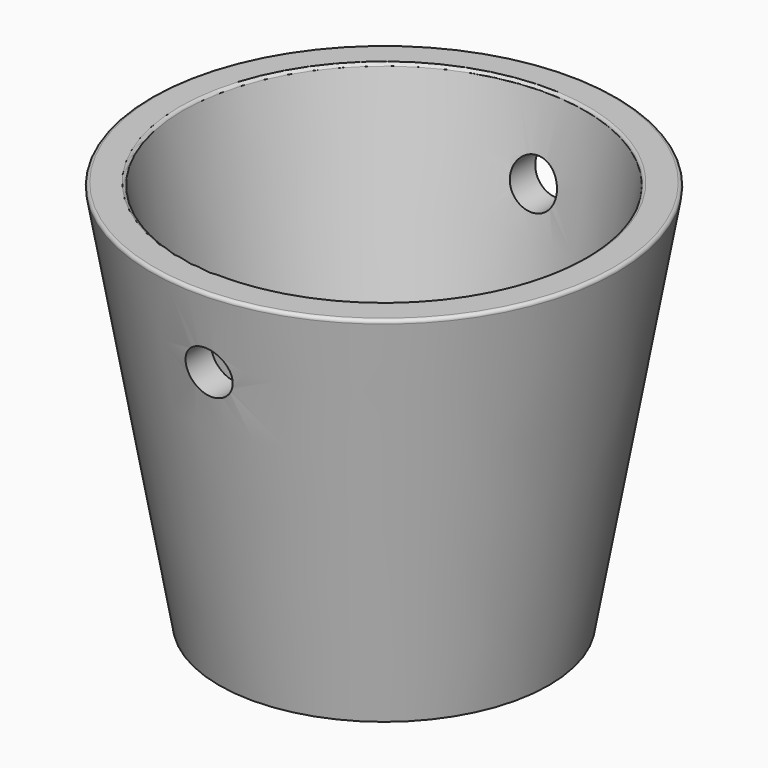
from build123d import *

# Parameters (mm, degrees)
F2_T          = -5.08
F3_R          = 3.81
F4_DEPTH      = 50.292
F4_DEPTH_BACK = 74.168
F5_R          = 0.508


with BuildPart() as f1:
    # F0 (on Front) → F1 (revolve)
    with BuildSketch(Plane.XZ):
        Polygon((0, 0), (0, 63.5), (-38.1, 63.5), (-26.903236725, 0), align=None)
    revolve(axis=Axis((0, 0, 31.75), (0, 0, 1)))

    # F2
    f2_openings = [f1.faces().sort_by_distance(p)[0] for p in [
        (0, 0, 63.5),
    ]]
    offset(amount=F2_T, openings=f2_openings)

    # F3 (on Front) → F4 (cut, two sides)
    with BuildSketch(Plane.XZ) as f4_sk:
        with Locations((0, 50.8)):
            Circle(F3_R)
    extrude(amount=-F4_DEPTH, mode=Mode.SUBTRACT)
    extrude(f4_sk.sketch, amount=F4_DEPTH_BACK, mode=Mode.SUBTRACT)

    # F5
    f5_edges = [f1.edges().sort_by_distance(p)[0] for p in [
        (32.941633, 0, 63.5),
        (38.1, 0, 63.5),
    ]]
    fillet(f5_edges, radius=F5_R)


solid = f1.part
